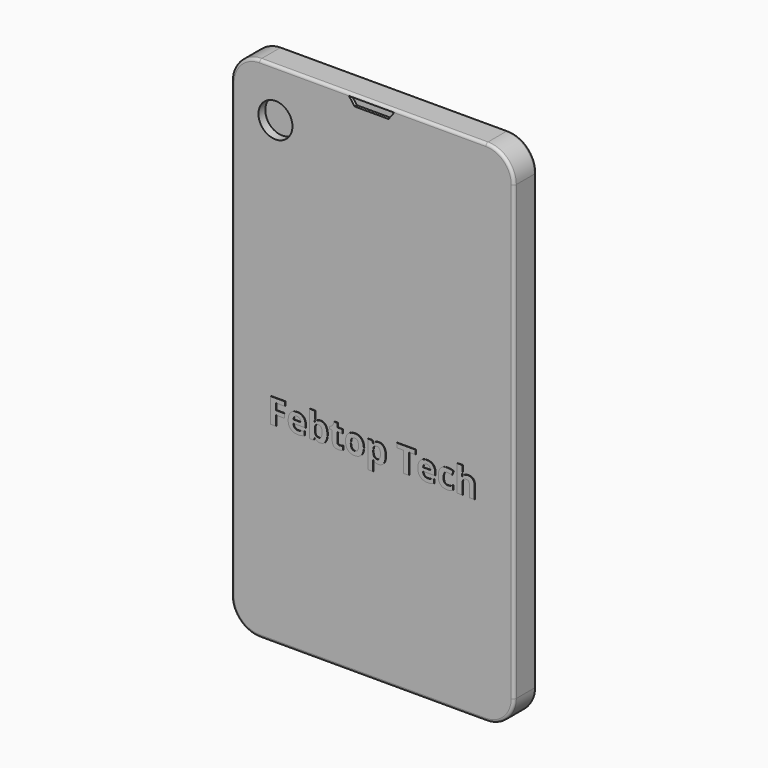
from build123d import *

# Parameters (mm, degrees)
F0_W          = 50
F0_H          = 90
F1_DEPTH      = 5
F2_R          = 5
F3_R          = 0.5
F4_R          = 0.5
F6_DEPTH      = 0.5
F7_R          = 3
F8_DEPTH      = 0.5
F9_DEPTH      = 1
F10_W         = 1.5
F10_H         = 17.8999968977
F11_DEPTH     = 1
F12_R         = 0.3
F13_TEXT_SIZE = 6.1163343321
F14_DEPTH     = 0.1


# Not quite as in the source:
# - Text() gives the source's letters only with a copy of the font that has no kerning and outlines rounded to 1/6400 em; it was checked with that copy


with BuildPart() as f1:
    # F0 (on Front) → F1 (new body)
    with BuildSketch(Plane.XZ):
        with Locations((0.1920731738, 3.2233093394)):
            Rectangle(F0_W, F0_H)
    extrude(amount=F1_DEPTH)

    # F2
    f2_edges = [f1.edges().sort_by_distance(p)[0] for p in [
        (-24.807927, -2.5, 48.223309),
        (25.192073, -2.5, 48.223309),
        (-24.807927, -2.5, -41.776691),
        (25.192073, -2.5, -41.776691),
    ]]
    fillet(f2_edges, radius=F2_R)

    # F3
    f3_edges = [f1.edges().sort_by_distance(p)[0] for p in [
        (-24.807927, -5, 3.223309),
        (-23.343461, -5, 46.758843),
        (0.192073, -5, 48.223309),
        (23.727607, -5, 46.758843),
        (25.192073, -5, 3.223309),
        (23.727607, -5, -40.312225),
        (0.192073, -5, -41.776691),
        (-23.343461, -5, -40.312225),
    ]]
    fillet(f3_edges, radius=F3_R)

    # F4
    f4_edges = [f1.edges().sort_by_distance(p)[0] for p in [
        (23.727607, 0, 46.758843),
        (0.192073, 0, 48.223309),
        (-23.343461, 0, 46.758843),
        (-24.807927, 0, 3.223309),
        (-23.343461, 0, -40.312225),
        (0.192073, 0, -41.776691),
        (23.727607, 0, -40.312225),
        (25.192073, 0, 3.223309),
    ]]
    fillet(f4_edges, radius=F4_R)

    # F5 (on face) → F6 (cut)
    with BuildSketch(Plane.XZ.offset(5)):
        Polygon((4, 47.7233093394), (-4, 47.7233093394), (-3, 46.3989786804), (3, 46.3989786804), align=None)
    extrude(amount=-F6_DEPTH, mode=Mode.SUBTRACT)

    # F7 (on face) → F8 (cut)
    with BuildSketch(Plane.XZ.offset(5)):
        with Locations((-17.0028377324, 39.7233093394)):
            Circle(F7_R)
    extrude(amount=-F8_DEPTH, mode=Mode.SUBTRACT)

    # F9 (cut): a face of the model
    f9_faces = [f1.faces().sort_by_distance(p)[0] for p in [
        (-17.0028377324, -4.5, 39.7233093394),
    ]]
    extrude(f9_faces, amount=-F9_DEPTH, mode=Mode.SUBTRACT)


with BuildPart() as f11:
    # F10 (on face) → F11 (new body)
    with BuildSketch(Plane(origin=(-24.8079268262, 0, 0), x_dir=(0, -1, 0), z_dir=(-1, 0, 0))):
        with Locations((2.5, 23.9253137261)):
            Rectangle(F10_W, F10_H)
    extrude(amount=F11_DEPTH)

    # F12
    f12_edges = [f11.edges().sort_by_distance(p)[0] for p in [
        (-25.807927, -3.25, 23.925314),
        (-25.807927, -1.75, 23.925314),
        (-25.807927, -2.5, 14.975315),
        (-25.807927, -2.5, 32.875312),
    ]]
    fillet(f12_edges, radius=F12_R)


with BuildPart() as f14:
    # F13 (on face) → F14 (new body)
    with BuildSketch(Plane.XZ.offset(5)):
        with Locations((-18.3079268262, -7.8274379289)):
            Text('Febtop Tech', F13_TEXT_SIZE, font='Open Sans', font_style=FontStyle.BOLD, text_align=(TextAlign.LEFT, TextAlign.BOTTOM))
    extrude(amount=F14_DEPTH)


solid = Compound([f1.part, f11.part, f14.part])
